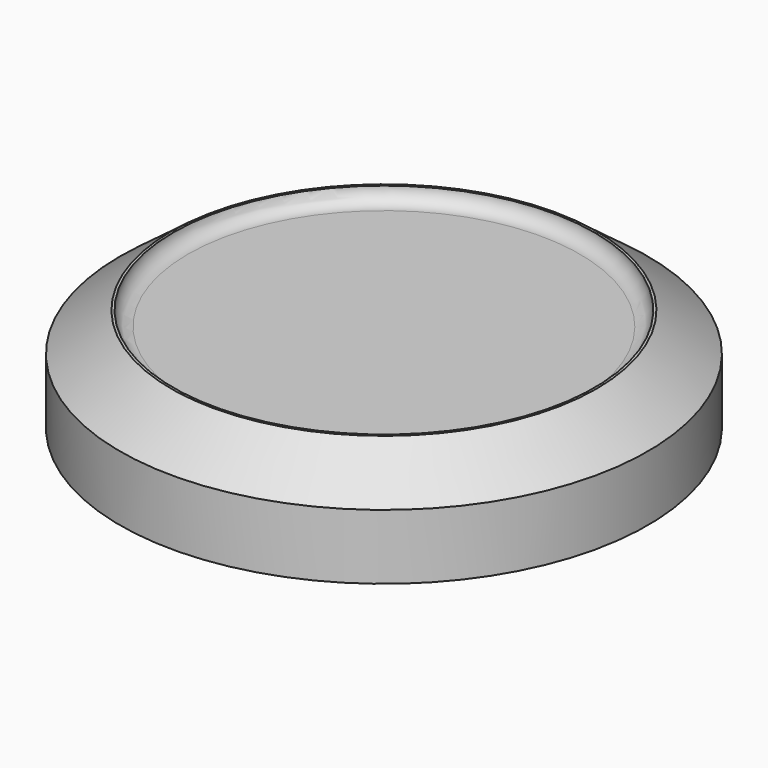
from build123d import *

# Parameters (mm, degrees)
F2_R = 5.99999


# Not quite as in the source:
# - a fillet or chamfer is up to 0.001 mm smaller than in the source, because OpenCascade refuses the exact size


with BuildPart() as f1:
    # F0 (on Front) → F1 (revolve)
    with BuildSketch(Plane.XZ):
        Polygon((-109.55, 0), (0, 0), (0, 37), (-87.33, 37), (-87.33, 43), (-88.33, 43), (-109.55, 27.0095830568), align=None)
    revolve(axis=Axis((0, 0, 18.5), (0, 0, 1)))

    # F2 (radius 6 in the source; OpenCascade refuses exactly that, so slightly less here)
    f2_edges = [f1.edges().sort_by_distance(p)[0] for p in [
        (87.33, 0, 37),
    ]]
    fillet(f2_edges, radius=F2_R)


solid = f1.part
